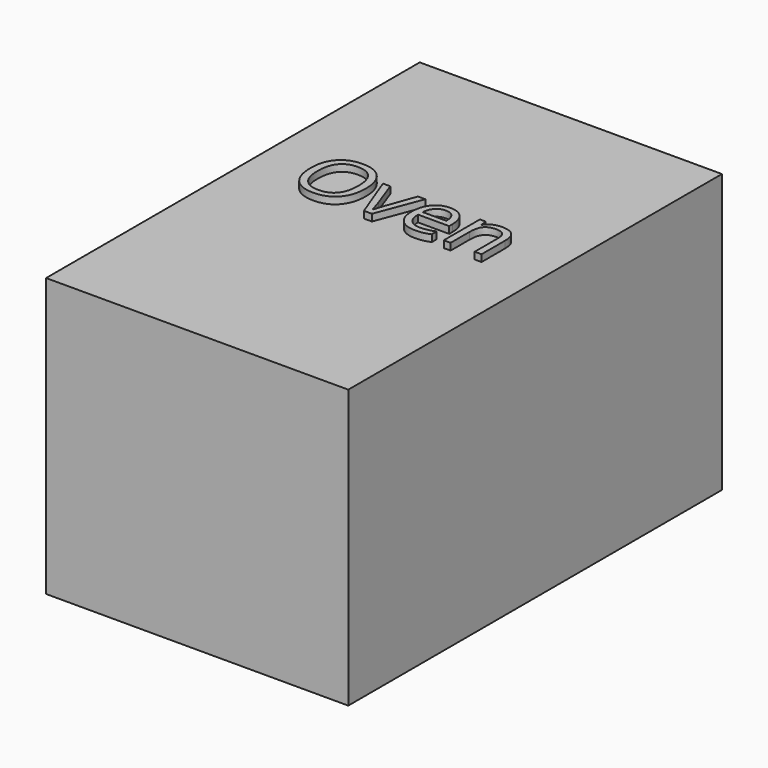
from build123d import *

# Parameters (mm, degrees)
F0_W         = 1117.6
F0_H         = 1727.2
F1_DEPTH     = 1028.7
F2_TEXT_SIZE = 312.4351335768
F3_DEPTH     = 25.4


# Not quite as in the source:
# - Text() gives the source's letters only with a copy of the font that has no kerning and outlines rounded to 1/6400 em; it was checked with that copy


with BuildPart() as f1:
    # F0 (on Top) → F1 (new body)
    with BuildSketch(Plane.XY):
        Rectangle(F0_W, F0_H)
    extrude(amount=F1_DEPTH)

    # F2 (on face) → F3 (join)
    with BuildSketch(Plane.XY.offset(1028.7)):
        with Locations((-381, 0)):
            Text('Oven', F2_TEXT_SIZE, font='Open Sans', text_align=(TextAlign.LEFT, TextAlign.BOTTOM))
    extrude(amount=F3_DEPTH)


solid = f1.part
